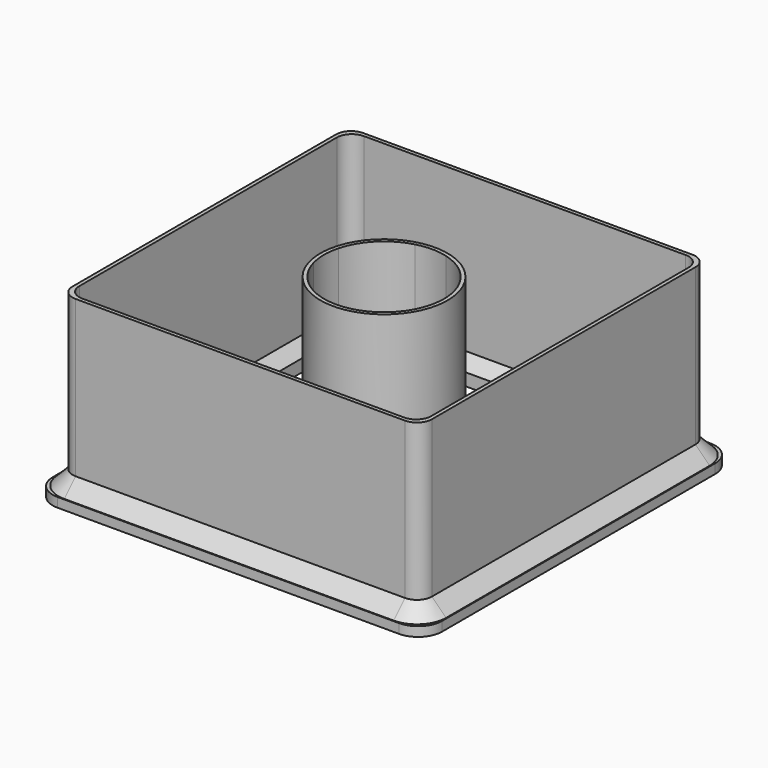
from build123d import *

# Parameters (mm, degrees)
F0_W          = 82.55
F0_H          = 82.55
F0_R          = 4.7625
F1_DEPTH      = 2
F2_DEPTH      = 38.1
F3_R          = 5.08
F4_T4_DEPTH   = 68.2625
F4_T10_DEPTH  = 68.2625
F4_T16_DEPTH  = 68.2625
F4_T23_DEPTH  = 68.2625
F4_T29_DEPTH  = 68.2625
F4_T35_DEPTH  = 68.2625
F4_T41_DEPTH  = 68.2625
F4_T47_DEPTH  = 68.2625
F4_T54_DEPTH  = 68.2625
F4_T60_DEPTH  = 68.2625
F4_T66_DEPTH  = 68.2625
F4_T72_DEPTH  = 68.2625
F4_T78_DEPTH  = 68.2625
F4_T85_DEPTH  = 68.2625
F4_T91_DEPTH  = 68.2625
F4_T97_DEPTH  = 68.2625
F4_T103_DEPTH = 68.2625
F4_T109_DEPTH = 68.2625
F4_T116_DEPTH = 68.2625
F4_T122_DEPTH = 68.2625
F4_T128_ANGLE = 121.67291642
F4_T134_ANGLE = 121.67291642
F4_T140_ANGLE = 121.67291642
F4_T146_ANGLE = 121.67291642
F4_T150_ANGLE = 90
F4_T152_ANGLE = 90
F4_T154_ANGLE = 90
F4_T156_ANGLE = 90
F5_SIZE       = 3
F6_SIZE       = 2.9972


# Not quite as in the source:
# - a fillet or chamfer that OpenCascade refuses, or shapes differently, is made with other operations: its cross-section is extruded or revolved along the edge and cut away or added


with BuildPart() as f1:
    # F0 (on Top) → F1 (new body)
    with BuildSketch(Plane.XY):
        Rectangle(F0_W, F0_H)
        with BuildLine():
            ThreePointArc((-38.1, 34.925), (-37.1700640303, 37.1700640303), (-34.925, 38.1))
            Line((-34.925, 38.1), (34.925, 38.1))
            ThreePointArc((34.925, 38.1), (37.1700640303, 37.1700640303), (38.1, 34.925))
            Line((38.1, 34.925), (38.1, -34.925))
            ThreePointArc((38.1, -34.925), (37.1700640303, -37.1700640303), (34.925, -38.1))
            Line((34.925, -38.1), (-34.925, -38.1))
            ThreePointArc((-34.925, -38.1), (-37.1700640303, -37.1700640303), (-38.1, -34.925))
            Line((-38.1, -34.925), (-38.1, 34.925))
        make_face(mode=Mode.SUBTRACT)
        with BuildLine():
            Line((34.925, 38.1), (-34.925, 38.1))
            ThreePointArc((-34.925, 38.1), (-37.1700640303, 37.1700640303), (-38.1, 34.925))
            Line((-38.1, 34.925), (-38.1, -34.925))
            ThreePointArc((-38.1, -34.925), (-37.1700640303, -37.1700640303), (-34.925, -38.1))
            Line((-34.925, -38.1), (34.925, -38.1))
            ThreePointArc((34.925, -38.1), (37.1700640303, -37.1700640303), (38.1, -34.925))
            Line((38.1, -34.925), (38.1, 34.925))
            ThreePointArc((38.1, 34.925), (37.1700640303, 37.1700640303), (34.925, 38.1))
        make_face()
        with BuildLine():
            Line((-37.30625, -34.13125), (-37.30625, 34.13125))
            ThreePointArc((-37.30625, 34.13125), (-36.3763140303, 36.3763140303), (-34.13125, 37.30625))
            Line((-34.13125, 37.30625), (34.13125, 37.30625))
            ThreePointArc((34.13125, 37.30625), (36.3763140303, 36.3763140303), (37.30625, 34.13125))
            Line((37.30625, 34.13125), (37.30625, -34.13125))
            ThreePointArc((37.30625, -34.13125), (36.3763140303, -36.3763140303), (34.13125, -37.30625))
            Line((34.13125, -37.30625), (-34.13125, -37.30625))
            ThreePointArc((-34.13125, -37.30625), (-36.3763140303, -36.3763140303), (-37.30625, -34.13125))
        make_face(mode=Mode.SUBTRACT)
        with BuildLine():
            ThreePointArc((-34.13125, 37.30625), (-36.3763140303, 36.3763140303), (-37.30625, 34.13125))
            Line((-37.30625, 34.13125), (-37.30625, -34.13125))
            ThreePointArc((-37.30625, -34.13125), (-36.3763140303, -36.3763140303), (-34.13125, -37.30625))
            Line((-34.13125, -37.30625), (34.13125, -37.30625))
            ThreePointArc((34.13125, -37.30625), (36.3763140303, -36.3763140303), (37.30625, -34.13125))
            Line((37.30625, -34.13125), (37.30625, 34.13125))
            ThreePointArc((37.30625, 34.13125), (36.3763140303, 36.3763140303), (34.13125, 37.30625))
            Line((34.13125, 37.30625), (-34.13125, 37.30625))
        make_face()
        Polygon((34.925, 34.925), (34.925, 25.9447438789), (34.925, -25.9447438789), (34.925, -34.925), (25.9447438789, -34.925), (-25.9447438789, -34.925), (-34.925, -34.925), (-34.925, -25.9447438789), (-34.925, 25.9447438789), (-34.925, 34.925), (-25.9447438789, 34.925), (25.9447438789, 34.925), align=None, mode=Mode.SUBTRACT)
        with BuildLine():
            Line((34.925, -25.9447438789), (12.909118174, -3.928862053))
            ThreePointArc((12.909118174, -3.928862053), (9.5415221286, -9.5415221286), (3.928862053, -12.909118174))
            Line((3.928862053, -12.909118174), (25.9447438789, -34.925))
            Line((25.9447438789, -34.925), (34.925, -34.925))
            Line((34.925, -34.925), (34.925, -25.9447438789))
        make_face()
        with BuildLine():
            ThreePointArc((-12.909118174, 3.928862053), (-9.5415221286, 9.5415221286), (-3.928862053, 12.909118174))
            Line((-3.928862053, 12.909118174), (-25.9447438789, 34.925))
            Line((-25.9447438789, 34.925), (-34.925, 34.925))
            Line((-34.925, 34.925), (-34.925, 25.9447438789))
            Line((-34.925, 25.9447438789), (-12.909118174, 3.928862053))
        make_face()
        with BuildLine():
            Line((-25.9447438789, -34.925), (-3.928862053, -12.909118174))
            ThreePointArc((-3.928862053, -12.909118174), (-9.5415221286, -9.5415221286), (-12.909118174, -3.928862053))
            Line((-12.909118174, -3.928862053), (-34.925, -25.9447438789))
            Line((-34.925, -25.9447438789), (-34.925, -34.925))
            Line((-34.925, -34.925), (-25.9447438789, -34.925))
        make_face()
        with BuildLine():
            ThreePointArc((3.928862053, 12.909118174), (9.5415221286, 9.5415221286), (12.909118174, 3.928862053))
            Line((12.909118174, 3.928862053), (34.925, 25.9447438789))
            Line((34.925, 25.9447438789), (34.925, 34.925))
            Line((34.925, 34.925), (25.9447438789, 34.925))
            Line((25.9447438789, 34.925), (3.928862053, 12.909118174))
        make_face()
        Polygon((0, -8.9802561211), (8.9802561211, 0), (0, 8.9802561211), (-8.9802561211, 0), align=None)
        Circle(F0_R, mode=Mode.SUBTRACT)
        with BuildLine():
            Line((0, 8.9802561211), (-3.2870018728, 12.2672579939))
            ThreePointArc((-3.2870018728, 12.2672579939), (-8.9802561211, 8.9802561211), (-12.2672579939, 3.2870018728))
            Line((-12.2672579939, 3.2870018728), (-8.9802561211, 0))
            Line((-8.9802561211, 0), (0, 8.9802561211))
        make_face()
        with BuildLine():
            Line((-3.2870018728, -12.2672579939), (0, -8.9802561211))
            Line((0, -8.9802561211), (-8.9802561211, 0))
            Line((-8.9802561211, 0), (-12.2672579939, -3.2870018728))
            ThreePointArc((-12.2672579939, -3.2870018728), (-8.9802561211, -8.9802561211), (-3.2870018728, -12.2672579939))
        make_face()
        with BuildLine():
            Line((8.9802561211, 0), (12.2672579939, 3.2870018728))
            ThreePointArc((12.2672579939, 3.2870018728), (8.9802561211, 8.9802561211), (3.2870018728, 12.2672579939))
            Line((3.2870018728, 12.2672579939), (0, 8.9802561211))
            Line((0, 8.9802561211), (8.9802561211, 0))
        make_face()
        with BuildLine():
            ThreePointArc((3.2870018728, -12.2672579939), (8.9802561211, -8.9802561211), (12.2672579939, -3.2870018728))
            Line((12.2672579939, -3.2870018728), (8.9802561211, 0))
            Line((8.9802561211, 0), (0, -8.9802561211))
            Line((0, -8.9802561211), (3.2870018728, -12.2672579939))
        make_face()
        with BuildLine():
            Line((-8.9802561211, 0), (-12.2672579939, 3.2870018728))
            ThreePointArc((-12.2672579939, 3.2870018728), (-12.7, 0), (-12.2672579939, -3.2870018728))
            Line((-12.2672579939, -3.2870018728), (-8.9802561211, 0))
        make_face()
        with BuildLine():
            Line((0, 8.9802561211), (3.2870018728, 12.2672579939))
            ThreePointArc((3.2870018728, 12.2672579939), (0, 12.7), (-3.2870018728, 12.2672579939))
            Line((-3.2870018728, 12.2672579939), (0, 8.9802561211))
        make_face()
        with BuildLine():
            ThreePointArc((12.2672579939, -3.2870018728), (12.5913497394, -1.6576826412), (12.7, 0))
            ThreePointArc((12.7, 0), (12.5913497394, 1.6576826412), (12.2672579939, 3.2870018728))
            Line((12.2672579939, 3.2870018728), (8.9802561211, 0))
            Line((8.9802561211, 0), (12.2672579939, -3.2870018728))
        make_face()
        with BuildLine():
            ThreePointArc((-3.2870018728, -12.2672579939), (0, -12.7), (3.2870018728, -12.2672579939))
            Line((3.2870018728, -12.2672579939), (0, -8.9802561211))
            Line((0, -8.9802561211), (-3.2870018728, -12.2672579939))
        make_face()
        with BuildLine():
            Line((12.909118174, -3.928862053), (12.2672579939, -3.2870018728))
            ThreePointArc((12.2672579939, -3.2870018728), (8.9802561211, -8.9802561211), (3.2870018728, -12.2672579939))
            Line((3.2870018728, -12.2672579939), (3.928862053, -12.909118174))
            ThreePointArc((3.928862053, -12.909118174), (9.5415221286, -9.5415221286), (12.909118174, -3.928862053))
        make_face()
        with BuildLine():
            ThreePointArc((-12.2672579939, 3.2870018728), (-8.9802561211, 8.9802561211), (-3.2870018728, 12.2672579939))
            Line((-3.2870018728, 12.2672579939), (-3.928862053, 12.909118174))
            ThreePointArc((-3.928862053, 12.909118174), (-9.5415221286, 9.5415221286), (-12.909118174, 3.928862053))
            Line((-12.909118174, 3.928862053), (-12.2672579939, 3.2870018728))
        make_face()
        with BuildLine():
            ThreePointArc((3.2870018728, 12.2672579939), (8.9802561211, 8.9802561211), (12.2672579939, 3.2870018728))
            Line((12.2672579939, 3.2870018728), (12.909118174, 3.928862053))
            ThreePointArc((12.909118174, 3.928862053), (9.5415221286, 9.5415221286), (3.928862053, 12.909118174))
            Line((3.928862053, 12.909118174), (3.2870018728, 12.2672579939))
        make_face()
        with BuildLine():
            Line((-3.928862053, -12.909118174), (-3.2870018728, -12.2672579939))
            ThreePointArc((-3.2870018728, -12.2672579939), (-8.9802561211, -8.9802561211), (-12.2672579939, -3.2870018728))
            Line((-12.2672579939, -3.2870018728), (-12.909118174, -3.928862053))
            ThreePointArc((-12.909118174, -3.928862053), (-9.5415221286, -9.5415221286), (-3.928862053, -12.909118174))
        make_face()
        with BuildLine():
            ThreePointArc((-3.2870018728, 12.2672579939), (0, 12.7), (3.2870018728, 12.2672579939))
            Line((3.2870018728, 12.2672579939), (3.928862053, 12.909118174))
            ThreePointArc((3.928862053, 12.909118174), (0, 13.49375), (-3.928862053, 12.909118174))
            Line((-3.928862053, 12.909118174), (-3.2870018728, 12.2672579939))
        make_face()
        with BuildLine():
            ThreePointArc((-12.2672579939, -3.2870018728), (-12.7, 0), (-12.2672579939, 3.2870018728))
            Line((-12.2672579939, 3.2870018728), (-12.909118174, 3.928862053))
            ThreePointArc((-12.909118174, 3.928862053), (-13.49375, 0), (-12.909118174, -3.928862053))
            Line((-12.909118174, -3.928862053), (-12.2672579939, -3.2870018728))
        make_face()
        with BuildLine():
            Line((3.928862053, -12.909118174), (3.2870018728, -12.2672579939))
            ThreePointArc((3.2870018728, -12.2672579939), (0, -12.7), (-3.2870018728, -12.2672579939))
            Line((-3.2870018728, -12.2672579939), (-3.928862053, -12.909118174))
            ThreePointArc((-3.928862053, -12.909118174), (0, -13.49375), (3.928862053, -12.909118174))
        make_face()
        with BuildLine():
            ThreePointArc((12.2672579939, 3.2870018728), (12.5913497394, 1.6576826412), (12.7, 0))
            ThreePointArc((12.7, 0), (12.5913497394, -1.6576826412), (12.2672579939, -3.2870018728))
            Line((12.2672579939, -3.2870018728), (12.909118174, -3.928862053))
            ThreePointArc((12.909118174, -3.928862053), (13.3467917947, -1.986060888), (13.49375, 0))
            ThreePointArc((13.49375, 0), (13.3467917947, 1.986060888), (12.909118174, 3.928862053))
            Line((12.909118174, 3.928862053), (12.2672579939, 3.2870018728))
        make_face()
    extrude(amount=F1_DEPTH)

    # F0 (on Top) → F2 (join)
    with BuildSketch(Plane.XY):
        with BuildLine():
            Line((34.925, 38.1), (-34.925, 38.1))
            ThreePointArc((-34.925, 38.1), (-37.1700640303, 37.1700640303), (-38.1, 34.925))
            Line((-38.1, 34.925), (-38.1, -34.925))
            ThreePointArc((-38.1, -34.925), (-37.1700640303, -37.1700640303), (-34.925, -38.1))
            Line((-34.925, -38.1), (34.925, -38.1))
            ThreePointArc((34.925, -38.1), (37.1700640303, -37.1700640303), (38.1, -34.925))
            Line((38.1, -34.925), (38.1, 34.925))
            ThreePointArc((38.1, 34.925), (37.1700640303, 37.1700640303), (34.925, 38.1))
        make_face()
        with BuildLine():
            Line((-37.30625, -34.13125), (-37.30625, 34.13125))
            ThreePointArc((-37.30625, 34.13125), (-36.3763140303, 36.3763140303), (-34.13125, 37.30625))
            Line((-34.13125, 37.30625), (34.13125, 37.30625))
            ThreePointArc((34.13125, 37.30625), (36.3763140303, 36.3763140303), (37.30625, 34.13125))
            Line((37.30625, 34.13125), (37.30625, -34.13125))
            ThreePointArc((37.30625, -34.13125), (36.3763140303, -36.3763140303), (34.13125, -37.30625))
            Line((34.13125, -37.30625), (-34.13125, -37.30625))
            ThreePointArc((-34.13125, -37.30625), (-36.3763140303, -36.3763140303), (-37.30625, -34.13125))
        make_face(mode=Mode.SUBTRACT)
        with BuildLine():
            ThreePointArc((-12.2672579939, -3.2870018728), (-12.7, 0), (-12.2672579939, 3.2870018728))
            Line((-12.2672579939, 3.2870018728), (-12.909118174, 3.928862053))
            ThreePointArc((-12.909118174, 3.928862053), (-13.49375, 0), (-12.909118174, -3.928862053))
            Line((-12.909118174, -3.928862053), (-12.2672579939, -3.2870018728))
        make_face()
        with BuildLine():
            Line((12.909118174, -3.928862053), (12.2672579939, -3.2870018728))
            ThreePointArc((12.2672579939, -3.2870018728), (8.9802561211, -8.9802561211), (3.2870018728, -12.2672579939))
            Line((3.2870018728, -12.2672579939), (3.928862053, -12.909118174))
            ThreePointArc((3.928862053, -12.909118174), (9.5415221286, -9.5415221286), (12.909118174, -3.928862053))
        make_face()
        with BuildLine():
            ThreePointArc((-3.2870018728, 12.2672579939), (0, 12.7), (3.2870018728, 12.2672579939))
            Line((3.2870018728, 12.2672579939), (3.928862053, 12.909118174))
            ThreePointArc((3.928862053, 12.909118174), (0, 13.49375), (-3.928862053, 12.909118174))
            Line((-3.928862053, 12.909118174), (-3.2870018728, 12.2672579939))
        make_face()
        with BuildLine():
            ThreePointArc((-12.2672579939, 3.2870018728), (-8.9802561211, 8.9802561211), (-3.2870018728, 12.2672579939))
            Line((-3.2870018728, 12.2672579939), (-3.928862053, 12.909118174))
            ThreePointArc((-3.928862053, 12.909118174), (-9.5415221286, 9.5415221286), (-12.909118174, 3.928862053))
            Line((-12.909118174, 3.928862053), (-12.2672579939, 3.2870018728))
        make_face()
        with BuildLine():
            Line((-3.928862053, -12.909118174), (-3.2870018728, -12.2672579939))
            ThreePointArc((-3.2870018728, -12.2672579939), (-8.9802561211, -8.9802561211), (-12.2672579939, -3.2870018728))
            Line((-12.2672579939, -3.2870018728), (-12.909118174, -3.928862053))
            ThreePointArc((-12.909118174, -3.928862053), (-9.5415221286, -9.5415221286), (-3.928862053, -12.909118174))
        make_face()
        with BuildLine():
            Line((3.928862053, -12.909118174), (3.2870018728, -12.2672579939))
            ThreePointArc((3.2870018728, -12.2672579939), (0, -12.7), (-3.2870018728, -12.2672579939))
            Line((-3.2870018728, -12.2672579939), (-3.928862053, -12.909118174))
            ThreePointArc((-3.928862053, -12.909118174), (0, -13.49375), (3.928862053, -12.909118174))
        make_face()
        with BuildLine():
            ThreePointArc((12.2672579939, 3.2870018728), (12.5913497394, 1.6576826412), (12.7, 0))
            ThreePointArc((12.7, 0), (12.5913497394, -1.6576826412), (12.2672579939, -3.2870018728))
            Line((12.2672579939, -3.2870018728), (12.909118174, -3.928862053))
            ThreePointArc((12.909118174, -3.928862053), (13.3467917947, -1.986060888), (13.49375, 0))
            ThreePointArc((13.49375, 0), (13.3467917947, 1.986060888), (12.909118174, 3.928862053))
            Line((12.909118174, 3.928862053), (12.2672579939, 3.2870018728))
        make_face()
        with BuildLine():
            ThreePointArc((3.2870018728, 12.2672579939), (8.9802561211, 8.9802561211), (12.2672579939, 3.2870018728))
            Line((12.2672579939, 3.2870018728), (12.909118174, 3.928862053))
            ThreePointArc((12.909118174, 3.928862053), (9.5415221286, 9.5415221286), (3.928862053, 12.909118174))
            Line((3.928862053, 12.909118174), (3.2870018728, 12.2672579939))
        make_face()
    extrude(amount=F2_DEPTH)

    # F3
    f3_edges = [f1.edges().sort_by_distance(p)[0] for p in [
        (41.275, 41.275, 1),
        (41.275, -41.275, 1),
        (-41.275, -41.275, 1),
        (-41.275, 41.275, 1),
    ]]
    fillet(f3_edges, radius=F3_R)

    # F4: chamfer of 3 on 8 edges, made by hand


with BuildPart() as f4_tool2:
    # F4_s3 → F4_t4 (new body)
    with BuildSketch(Plane.XZ.offset(-34.13125)):
        Polygon((-34.30625, 2), (-37.30625, 5), (-37.30625, 2), align=None)
    extrude(amount=F4_T4_DEPTH)

    split(bisect_by=Plane(origin=(-4.4901280605, -4.4901280605, 0), x_dir=(0, 0, 1), z_dir=(0.7071067812, 0.7071067812, 0)), keep=Keep.TOP)

    split(bisect_by=Plane.YZ.offset(-34.925), keep=Keep.TOP)


with BuildPart() as f1_1:
    add(f1.part)

    # F4_t1: union F4_tool2
    add(f4_tool2.part)


with BuildPart() as f4_tool8:
    # F4_s9 → F4_t10 (new body)
    with BuildSketch(Plane.XZ.offset(-34.13125)):
        Polygon((-34.30625, 2), (-37.30625, 5), (-37.30625, 2), align=None)
    extrude(amount=F4_T10_DEPTH)

    split(bisect_by=Plane(origin=(-4.4901280605, -4.4901280605, 0), x_dir=(0, 0, 1), z_dir=(0.7071067812, 0.7071067812, 0)), keep=Keep.TOP)

    split(bisect_by=Plane.YZ.offset(-34.925), keep=Keep.BOTTOM)


with BuildPart() as f1_2:
    add(f1_1.part)

    # F4_t7: union F4_tool8
    add(f4_tool8.part)


with BuildPart() as f4_tool14:
    # F4_s15 → F4_t16 (new body)
    with BuildSketch(Plane.XZ.offset(-34.13125)):
        Polygon((-34.30625, 2), (-37.30625, 5), (-37.30625, 2), align=None)
    extrude(amount=F4_T16_DEPTH)

    split(bisect_by=Plane(origin=(-4.4901280605, -4.4901280605, 0), x_dir=(0, 0, 1), z_dir=(-0.7071067812, -0.7071067812, 0)), keep=Keep.TOP)

    split(bisect_by=Plane(origin=(-4.4901280605, 4.4901280605, 0), x_dir=(0, 0, 1), z_dir=(-0.7071067812, 0.7071067812, 0)), keep=Keep.TOP)

    split(bisect_by=Plane.YZ.offset(-34.925), keep=Keep.BOTTOM)


with BuildPart() as f1_3:
    add(f1_2.part)

    # F4_t13: union F4_tool14
    add(f4_tool14.part)


with BuildPart() as f4_tool21:
    # F4_s22 → F4_t23 (new body)
    with BuildSketch(Plane.XZ.offset(-34.13125)):
        Polygon((-34.30625, 2), (-37.30625, 5), (-37.30625, 2), align=None)
    extrude(amount=F4_T23_DEPTH)

    split(bisect_by=Plane(origin=(-4.4901280605, 4.4901280605, 0), x_dir=(0, 0, 1), z_dir=(0.7071067812, -0.7071067812, 0)), keep=Keep.TOP)

    split(bisect_by=Plane.YZ.offset(-34.925), keep=Keep.TOP)


with BuildPart() as f1_4:
    add(f1_3.part)

    # F4_t20: union F4_tool21
    add(f4_tool21.part)


with BuildPart() as f4_tool27:
    # F4_s28 → F4_t29 (new body)
    with BuildSketch(Plane.XZ.offset(-34.13125)):
        Polygon((-34.30625, 2), (-37.30625, 5), (-37.30625, 2), align=None)
    extrude(amount=F4_T29_DEPTH)

    split(bisect_by=Plane(origin=(-4.4901280605, 4.4901280605, 0), x_dir=(0, 0, 1), z_dir=(0.7071067812, -0.7071067812, 0)), keep=Keep.TOP)

    split(bisect_by=Plane.YZ.offset(-34.925), keep=Keep.BOTTOM)


with BuildPart() as f1_5:
    add(f1_4.part)

    # F4_t26: union F4_tool27
    add(f4_tool27.part)


with BuildPart() as f4_tool33:
    # F4_s34 → F4_t35 (new body)
    with BuildSketch(Plane.YZ.offset(34.13125)):
        Polygon((34.30625, 2), (37.30625, 5), (37.30625, 2), align=None)
    extrude(amount=-F4_T35_DEPTH)

    split(bisect_by=Plane.XZ.offset(-34.925), keep=Keep.TOP)

    split(bisect_by=Plane(origin=(-4.4901280605, 4.4901280605, 0), x_dir=(0, 0, 1), z_dir=(0.7071067812, -0.7071067812, 0)), keep=Keep.TOP)


with BuildPart() as f1_6:
    add(f1_5.part)

    # F4_t32: union F4_tool33
    add(f4_tool33.part)


with BuildPart() as f4_tool39:
    # F4_s40 → F4_t41 (new body)
    with BuildSketch(Plane.YZ.offset(34.13125)):
        Polygon((34.30625, 2), (37.30625, 5), (37.30625, 2), align=None)
    extrude(amount=-F4_T41_DEPTH)

    split(bisect_by=Plane.XZ.offset(-34.925), keep=Keep.BOTTOM)

    split(bisect_by=Plane(origin=(-4.4901280605, 4.4901280605, 0), x_dir=(0, 0, 1), z_dir=(0.7071067812, -0.7071067812, 0)), keep=Keep.TOP)


with BuildPart() as f1_7:
    add(f1_6.part)

    # F4_t38: union F4_tool39
    add(f4_tool39.part)


with BuildPart() as f4_tool45:
    # F4_s46 → F4_t47 (new body)
    with BuildSketch(Plane.YZ.offset(34.13125)):
        Polygon((34.30625, 2), (37.30625, 5), (37.30625, 2), align=None)
    extrude(amount=-F4_T47_DEPTH)

    split(bisect_by=Plane.XZ.offset(-34.925), keep=Keep.BOTTOM)

    split(bisect_by=Plane(origin=(-4.4901280605, 4.4901280605, 0), x_dir=(0, 0, 1), z_dir=(-0.7071067812, 0.7071067812, 0)), keep=Keep.TOP)

    split(bisect_by=Plane(origin=(4.4901280605, 4.4901280605, 0), x_dir=(0, 0, 1), z_dir=(0.7071067812, 0.7071067812, 0)), keep=Keep.TOP)


with BuildPart() as f1_8:
    add(f1_7.part)

    # F4_t44: union F4_tool45
    add(f4_tool45.part)


with BuildPart() as f4_tool52:
    # F4_s53 → F4_t54 (new body)
    with BuildSketch(Plane.YZ.offset(34.13125)):
        Polygon((34.30625, 2), (37.30625, 5), (37.30625, 2), align=None)
    extrude(amount=-F4_T54_DEPTH)

    split(bisect_by=Plane.XZ.offset(-34.925), keep=Keep.TOP)

    split(bisect_by=Plane(origin=(4.4901280605, 4.4901280605, 0), x_dir=(0, 0, 1), z_dir=(-0.7071067812, -0.7071067812, 0)), keep=Keep.TOP)


with BuildPart() as f1_9:
    add(f1_8.part)

    # F4_t51: union F4_tool52
    add(f4_tool52.part)


with BuildPart() as f4_tool58:
    # F4_s59 → F4_t60 (new body)
    with BuildSketch(Plane.YZ.offset(34.13125)):
        Polygon((34.30625, 2), (37.30625, 5), (37.30625, 2), align=None)
    extrude(amount=-F4_T60_DEPTH)

    split(bisect_by=Plane.XZ.offset(-34.925), keep=Keep.BOTTOM)

    split(bisect_by=Plane(origin=(4.4901280605, 4.4901280605, 0), x_dir=(0, 0, 1), z_dir=(-0.7071067812, -0.7071067812, 0)), keep=Keep.TOP)


with BuildPart() as f1_10:
    add(f1_9.part)

    # F4_t57: union F4_tool58
    add(f4_tool58.part)


with BuildPart() as f4_tool64:
    # F4_s65 → F4_t66 (new body)
    with BuildSketch(Plane.XZ.offset(34.13125)):
        Polygon((34.30625, 2), (37.30625, 5), (37.30625, 2), align=None)
    extrude(amount=-F4_T66_DEPTH)

    split(bisect_by=Plane(origin=(4.4901280605, 4.4901280605, 0), x_dir=(0, 0, 1), z_dir=(-0.7071067812, -0.7071067812, 0)), keep=Keep.TOP)

    split(bisect_by=Plane.YZ.offset(34.925), keep=Keep.BOTTOM)


with BuildPart() as f1_11:
    add(f1_10.part)

    # F4_t63: union F4_tool64
    add(f4_tool64.part)


with BuildPart() as f4_tool70:
    # F4_s71 → F4_t72 (new body)
    with BuildSketch(Plane.XZ.offset(34.13125)):
        Polygon((34.30625, 2), (37.30625, 5), (37.30625, 2), align=None)
    extrude(amount=-F4_T72_DEPTH)

    split(bisect_by=Plane(origin=(4.4901280605, 4.4901280605, 0), x_dir=(0, 0, 1), z_dir=(-0.7071067812, -0.7071067812, 0)), keep=Keep.TOP)

    split(bisect_by=Plane.YZ.offset(34.925), keep=Keep.TOP)


with BuildPart() as f1_12:
    add(f1_11.part)

    # F4_t69: union F4_tool70
    add(f4_tool70.part)


with BuildPart() as f4_tool76:
    # F4_s77 → F4_t78 (new body)
    with BuildSketch(Plane.XZ.offset(34.13125)):
        Polygon((34.30625, 2), (37.30625, 5), (37.30625, 2), align=None)
    extrude(amount=-F4_T78_DEPTH)

    split(bisect_by=Plane(origin=(4.4901280605, 4.4901280605, 0), x_dir=(0, 0, 1), z_dir=(0.7071067812, 0.7071067812, 0)), keep=Keep.TOP)

    split(bisect_by=Plane(origin=(4.4901280605, -4.4901280605, 0), x_dir=(0, 0, 1), z_dir=(0.7071067812, -0.7071067812, 0)), keep=Keep.TOP)

    split(bisect_by=Plane.YZ.offset(34.925), keep=Keep.TOP)


with BuildPart() as f1_13:
    add(f1_12.part)

    # F4_t75: union F4_tool76
    add(f4_tool76.part)


with BuildPart() as f4_tool83:
    # F4_s84 → F4_t85 (new body)
    with BuildSketch(Plane.XZ.offset(34.13125)):
        Polygon((34.30625, 2), (37.30625, 5), (37.30625, 2), align=None)
    extrude(amount=-F4_T85_DEPTH)

    split(bisect_by=Plane(origin=(4.4901280605, -4.4901280605, 0), x_dir=(0, 0, 1), z_dir=(-0.7071067812, 0.7071067812, 0)), keep=Keep.TOP)

    split(bisect_by=Plane.YZ.offset(34.925), keep=Keep.BOTTOM)


with BuildPart() as f1_14:
    add(f1_13.part)

    # F4_t82: union F4_tool83
    add(f4_tool83.part)


with BuildPart() as f4_tool89:
    # F4_s90 → F4_t91 (new body)
    with BuildSketch(Plane.XZ.offset(34.13125)):
        Polygon((34.30625, 2), (37.30625, 5), (37.30625, 2), align=None)
    extrude(amount=-F4_T91_DEPTH)

    split(bisect_by=Plane(origin=(4.4901280605, -4.4901280605, 0), x_dir=(0, 0, 1), z_dir=(-0.7071067812, 0.7071067812, 0)), keep=Keep.TOP)

    split(bisect_by=Plane.YZ.offset(34.925), keep=Keep.TOP)


with BuildPart() as f1_15:
    add(f1_14.part)

    # F4_t88: union F4_tool89
    add(f4_tool89.part)


with BuildPart() as f4_tool95:
    # F4_s96 → F4_t97 (new body)
    with BuildSketch(Plane.YZ.offset(-34.13125)):
        Polygon((-34.30625, 2), (-37.30625, 5), (-37.30625, 2), align=None)
    extrude(amount=F4_T97_DEPTH)

    split(bisect_by=Plane(origin=(4.4901280605, -4.4901280605, 0), x_dir=(0, 0, 1), z_dir=(-0.7071067812, 0.7071067812, 0)), keep=Keep.TOP)

    split(bisect_by=Plane.XZ.offset(34.925), keep=Keep.BOTTOM)


with BuildPart() as f1_16:
    add(f1_15.part)

    # F4_t94: union F4_tool95
    add(f4_tool95.part)


with BuildPart() as f4_tool101:
    # F4_s102 → F4_t103 (new body)
    with BuildSketch(Plane.YZ.offset(-34.13125)):
        Polygon((-34.30625, 2), (-37.30625, 5), (-37.30625, 2), align=None)
    extrude(amount=F4_T103_DEPTH)

    split(bisect_by=Plane(origin=(4.4901280605, -4.4901280605, 0), x_dir=(0, 0, 1), z_dir=(-0.7071067812, 0.7071067812, 0)), keep=Keep.TOP)

    split(bisect_by=Plane.XZ.offset(34.925), keep=Keep.TOP)


with BuildPart() as f1_17:
    add(f1_16.part)

    # F4_t100: union F4_tool101
    add(f4_tool101.part)


with BuildPart() as f4_tool107:
    # F4_s108 → F4_t109 (new body)
    with BuildSketch(Plane.YZ.offset(-34.13125)):
        Polygon((-34.30625, 2), (-37.30625, 5), (-37.30625, 2), align=None)
    extrude(amount=F4_T109_DEPTH)

    split(bisect_by=Plane(origin=(4.4901280605, -4.4901280605, 0), x_dir=(0, 0, 1), z_dir=(0.7071067812, -0.7071067812, 0)), keep=Keep.TOP)

    split(bisect_by=Plane(origin=(-4.4901280605, -4.4901280605, 0), x_dir=(0, 0, 1), z_dir=(-0.7071067812, -0.7071067812, 0)), keep=Keep.TOP)

    split(bisect_by=Plane.XZ.offset(34.925), keep=Keep.TOP)


with BuildPart() as f1_18:
    add(f1_17.part)

    # F4_t106: union F4_tool107
    add(f4_tool107.part)


with BuildPart() as f4_tool114:
    # F4_s115 → F4_t116 (new body)
    with BuildSketch(Plane.YZ.offset(-34.13125)):
        Polygon((-34.30625, 2), (-37.30625, 5), (-37.30625, 2), align=None)
    extrude(amount=F4_T116_DEPTH)

    split(bisect_by=Plane(origin=(-4.4901280605, -4.4901280605, 0), x_dir=(0, 0, 1), z_dir=(0.7071067812, 0.7071067812, 0)), keep=Keep.TOP)

    split(bisect_by=Plane.XZ.offset(34.925), keep=Keep.BOTTOM)


with BuildPart() as f1_19:
    add(f1_18.part)

    # F4_t113: union F4_tool114
    add(f4_tool114.part)


with BuildPart() as f4_tool120:
    # F4_s121 → F4_t122 (new body)
    with BuildSketch(Plane.YZ.offset(-34.13125)):
        Polygon((-34.30625, 2), (-37.30625, 5), (-37.30625, 2), align=None)
    extrude(amount=F4_T122_DEPTH)

    split(bisect_by=Plane(origin=(-4.4901280605, -4.4901280605, 0), x_dir=(0, 0, 1), z_dir=(0.7071067812, 0.7071067812, 0)), keep=Keep.TOP)

    split(bisect_by=Plane.XZ.offset(34.925), keep=Keep.TOP)


with BuildPart() as f1_20:
    add(f1_19.part)

    # F4_t119: union F4_tool120
    add(f4_tool120.part)


with BuildPart() as f4_tool126:
    # F4_s127 → F4_t128 (revolve)
    with BuildSketch(Plane(origin=(0, 0, 0), x_dir=(0, 0, 1), z_dir=(-0.2728924664, 0.9620445425, 0))):
        Polygon((5, 13.49375), (2, 16.49375), (2, 13.49375), align=None)
    revolve(axis=Axis((0, 0, 2), (0, 0, -1)), revolution_arc=F4_T128_ANGLE)

    split(bisect_by=Plane(origin=(-4.4901280605, -4.4901280605, 0), x_dir=(0, 0, 1), z_dir=(0.7071067812, 0.7071067812, 0)), keep=Keep.TOP)

    split(bisect_by=Plane(origin=(4.4901280605, 4.4901280605, 0), x_dir=(0, 0, 1), z_dir=(-0.7071067812, -0.7071067812, 0)), keep=Keep.TOP)


with BuildPart() as f1_21:
    add(f1_20.part)

    # F4_t125: union F4_tool126
    add(f4_tool126.part)


with BuildPart() as f4_tool132:
    # F4_s133 → F4_t134 (revolve)
    with BuildSketch(Plane(origin=(0, 0, 0), x_dir=(0, 0, 1), z_dir=(-0.9620445425, -0.2728924664, 0))):
        Polygon((5, 13.49375), (2, 16.49375), (2, 13.49375), align=None)
    revolve(axis=Axis((0, 0, 2), (0, 0, -1)), revolution_arc=F4_T134_ANGLE)

    split(bisect_by=Plane(origin=(-4.4901280605, 4.4901280605, 0), x_dir=(0, 0, 1), z_dir=(0.7071067812, -0.7071067812, 0)), keep=Keep.TOP)

    split(bisect_by=Plane(origin=(4.4901280605, -4.4901280605, 0), x_dir=(0, 0, 1), z_dir=(-0.7071067812, 0.7071067812, 0)), keep=Keep.TOP)


with BuildPart() as f1_22:
    add(f1_21.part)

    # F4_t131: union F4_tool132
    add(f4_tool132.part)


with BuildPart() as f4_tool138:
    # F4_s139 → F4_t140 (revolve)
    with BuildSketch(Plane(origin=(0, 0, 0), x_dir=(0, 0, 1), z_dir=(0.2728924664, -0.9620445425, 0))):
        Polygon((5, 13.49375), (2, 16.49375), (2, 13.49375), align=None)
    revolve(axis=Axis((0, 0, 2), (0, 0, -1)), revolution_arc=F4_T140_ANGLE)

    split(bisect_by=Plane(origin=(4.4901280605, 4.4901280605, 0), x_dir=(0, 0, 1), z_dir=(-0.7071067812, -0.7071067812, 0)), keep=Keep.TOP)

    split(bisect_by=Plane(origin=(-4.4901280605, -4.4901280605, 0), x_dir=(0, 0, 1), z_dir=(0.7071067812, 0.7071067812, 0)), keep=Keep.TOP)


with BuildPart() as f1_23:
    add(f1_22.part)

    # F4_t137: union F4_tool138
    add(f4_tool138.part)


with BuildPart() as f4_tool144:
    # F4_s145 → F4_t146 (revolve)
    with BuildSketch(Plane(origin=(0, 0, 0), x_dir=(0, 0, 1), z_dir=(0.9620445425, 0.2728924664, 0))):
        Polygon((5, 13.49375), (2, 16.49375), (2, 13.49375), align=None)
    revolve(axis=Axis((0, 0, 2), (0, 0, -1)), revolution_arc=F4_T146_ANGLE)

    split(bisect_by=Plane(origin=(-4.4901280605, 4.4901280605, 0), x_dir=(0, 0, 1), z_dir=(0.7071067812, -0.7071067812, 0)), keep=Keep.TOP)

    split(bisect_by=Plane(origin=(4.4901280605, -4.4901280605, 0), x_dir=(0, 0, 1), z_dir=(-0.7071067812, 0.7071067812, 0)), keep=Keep.TOP)


with BuildPart() as f1_24:
    add(f1_23.part)

    # F4_t143: union F4_tool144
    add(f4_tool144.part)

    # F4_s149 → F4_t150 (revolve)
    with BuildSketch(Plane.YZ.offset(-34.13125)):
        Polygon((-34.30625, 2), (-37.30625, 5), (-37.30625, 2), align=None)
    revolve(axis=Axis((-34.13125, -34.13125, 2), (0, 0, -1)), revolution_arc=F4_T150_ANGLE)

    # F4_s151 → F4_t152 (revolve)
    with BuildSketch(Plane.XZ.offset(34.13125)):
        Polygon((34.30625, 2), (37.30625, 5), (37.30625, 2), align=None)
    revolve(axis=Axis((34.13125, -34.13125, 2), (0, 0, -1)), revolution_arc=F4_T152_ANGLE)

    # F4_s153 → F4_t154 (revolve)
    with BuildSketch(Plane.YZ.offset(34.13125)):
        Polygon((34.30625, 2), (37.30625, 5), (37.30625, 2), align=None)
    revolve(axis=Axis((34.13125, 34.13125, 2), (0, 0, -1)), revolution_arc=F4_T154_ANGLE)

    # F4_s155 → F4_t156 (revolve)
    with BuildSketch(Plane.XZ.offset(-34.13125)):
        Polygon((-34.30625, 2), (-37.30625, 5), (-37.30625, 2), align=None)
    revolve(axis=Axis((-34.13125, 34.13125, 2), (0, 0, -1)), revolution_arc=F4_T156_ANGLE)

    # F5
    f5_edges = [f1_24.edges().sort_by_distance(p)[0] for p in [
        (-38.1, 0, 2),
        (0, -38.1, 2),
        (38.1, 0, 2),
        (0, 38.1, 2),
    ]]
    chamfer(f5_edges, length=F5_SIZE)

    # F6
    f6_edges = [f1_24.edges().sort_by_distance(p)[0] for p in [
        (-3.287002, -12.267258, 2),
    ]]
    chamfer(f6_edges, length=F6_SIZE)


solid = f1_24.part
